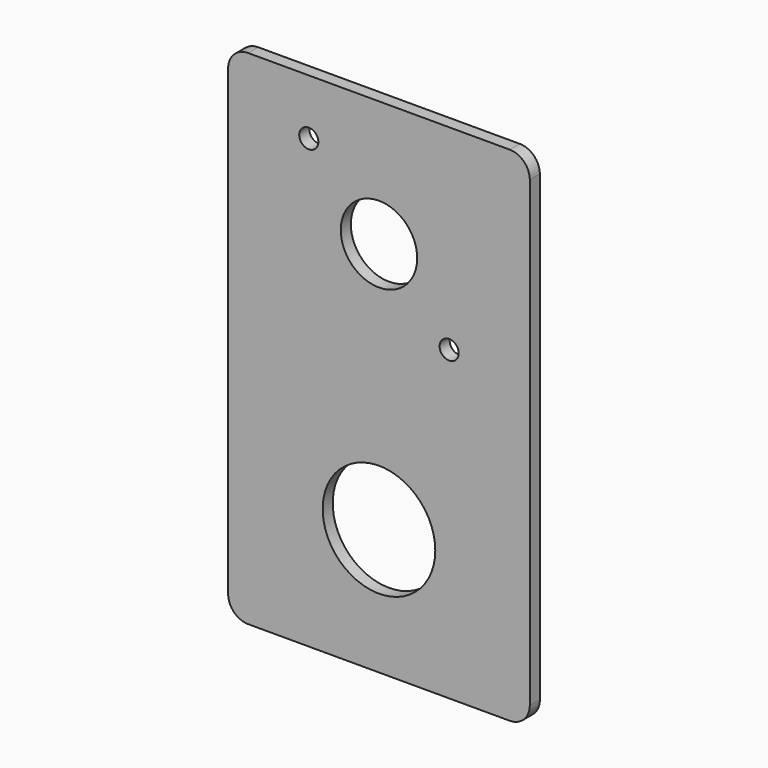
from build123d import *

# Parameters (mm, degrees)
F0_R     = 14.224
F0_R_2   = 2.413
F0_R_3   = 9.652
F1_DEPTH = 3.175
F2_R     = 5.08


# Not quite as in the source:
# - a length typed as a fraction of an inch, garbled in the dataset ("3 / 203.2 mm" for 3/8 in), is restored


with BuildPart() as f1:
    # F0 (on Front) → F1 (new body)
    with BuildSketch(Plane.XZ):
        Polygon((-38.1, -95.25), (38.1, -95.25), (38.1, -77.7618959546), (38.1, -65.0618959546), (38.1, 31.75), (-38.1, 31.75), align=None)
        with Locations((0, -63.5)):
            Circle(F0_R, mode=Mode.SUBTRACT)
        with Locations((-17.7292, 17.7292)):
            Circle(F0_R_2, mode=Mode.SUBTRACT)
        Circle(F0_R_3, mode=Mode.SUBTRACT)
        with Locations((17.7292, -17.7292)):
            Circle(F0_R_2, mode=Mode.SUBTRACT)
    extrude(amount=F1_DEPTH)

    # F2
    f2_edges = [f1.edges().sort_by_distance(p)[0] for p in [
        (38.1, -1.5875, -95.25),
        (38.1, -1.5875, 31.75),
        (-38.1, -1.5875, -95.25),
        (-38.1, -1.5875, 31.75),
    ]]
    fillet(f2_edges, radius=F2_R)


solid = f1.part
